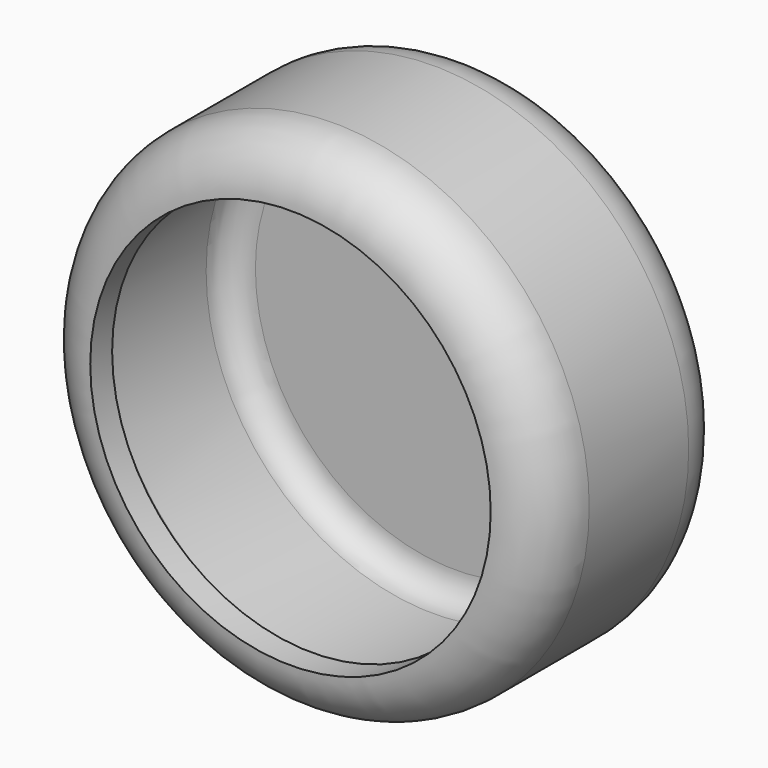
from build123d import *

# Parameters (mm, degrees)
F0_R     = 23.6631657712
F1_DEPTH = 21.69927
F2_R     = 5.08
F3_T     = -2.54


# Not quite as in the source:
# - a shell that OpenCascade refuses in one call is made with other operations: the cavity is built on its own and cut out


with BuildPart() as f1:
    # F0 (on Front) → F1 (new body)
    with BuildSketch(Plane.XZ):
        Circle(F0_R)
    extrude(amount=F1_DEPTH)

    # F2
    f2_edges = [f1.edges().sort_by_distance(p)[0] for p in [
        (-23.663166, -21.69927, 0),
        (-23.663166, 0, 0),
    ]]
    fillet(f2_edges, radius=F2_R)

    # F3: a shell. OpenCascade refuses it in one call, so the cavity is built on its own and cut out:
    # the body offset inwards by the wall thickness, plus a prism from it out through each open face.
    f3_core = offset(f1.part, amount=F3_T, mode=Mode.PRIVATE)
    f3_exits = [f3_core.faces().sort_by_distance(p)[0] for p in [
        (0, -19.15927, 0),
    ]]
    add(f3_core, mode=Mode.SUBTRACT)
    extrude(f3_exits, amount=-F3_T, mode=Mode.SUBTRACT)


solid = f1.part
